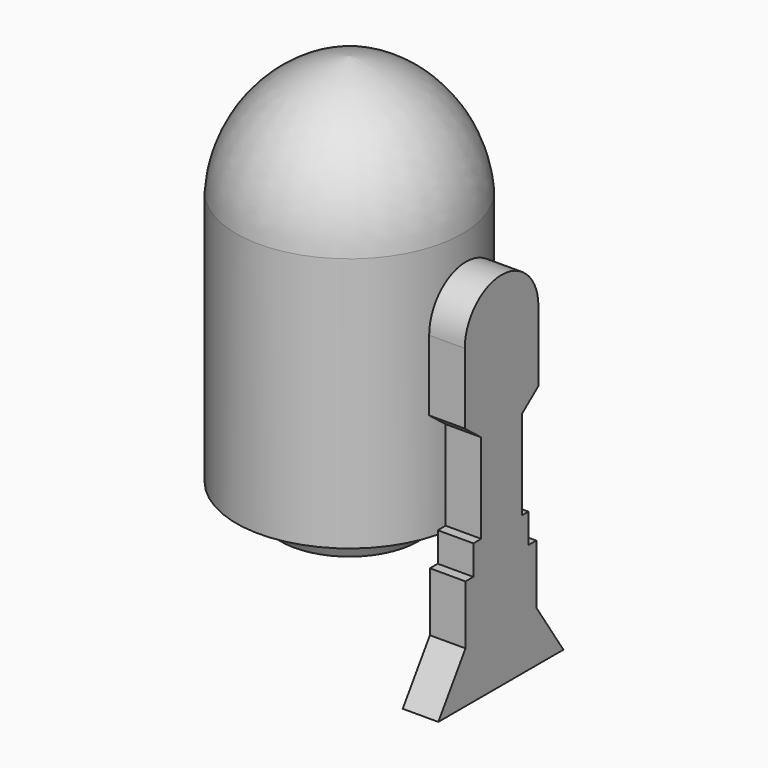
from build123d import *

# Parameters (mm, degrees)
F4_DEPTH = 8.8


with BuildPart() as f1:
    # F0 (on Front) → F1 (revolve)
    with BuildSketch(Plane.XZ):
        with BuildLine():
            ThreePointArc((27.9495026916, 0), (19.2278922615, 19.7592115619), (0, 29.5969495755))
            Line((0, 29.5969495755), (0, -70.4030504245))
            Line((0, -70.4030504245), (16.9765111059, -70.5251395702))
            Line((16.9765111059, -70.5251395702), (20.9008958191, -63.0331337452))
            Line((20.9008958191, -63.0331337452), (27.9495026916, -63.0331337452))
            Line((27.9495026916, -63.0331337452), (27.9495026916, 0))
        make_face()
    revolve(axis=Axis((0, 0, -20.4030504245), (0, 0, -1)))


with BuildPart() as f4:
    # F3 (on offset) → F4 (new body)
    with BuildSketch(Plane.YZ.offset(28)):
        with BuildLine():
            Line((-10.345963412, -17.8559850901), (-10.345963412, -35.3041645139))
            Line((-10.345963412, -35.3041645139), (-5.2661128575, -39.2796974629))
            Line((-5.2661128575, -39.2796974629), (-5.2661128575, -61.3659974188))
            Line((-5.2661128575, -61.3659974188), (-7.6956056291, -61.3659974188))
            Line((-7.6956056291, -61.3659974188), (-7.6956056291, -68.6544794589))
            Line((-7.6956056291, -68.6544794589), (-10.1250984007, -68.6544794589))
            Line((-10.1250984007, -68.6544794589), (-10.1250984007, -83.2314360887))
            Line((-10.1250984007, -83.2314360887), (-18.5178943211, -95.8206299692))
            Line((-18.5178943211, -95.8206299692), (20.1331399148, -95.8206299692))
            Line((20.1331399148, -95.8206299692), (11.7403439945, -83.2314360887))
            Line((11.7403439945, -83.2314360887), (11.7403439945, -68.6544794589))
            Line((11.7403439945, -68.6544794589), (9.3108512228, -68.6544794589))
            Line((9.3108512228, -68.6544794589), (9.3108512228, -61.3659974188))
            Line((9.3108512228, -61.3659974188), (7.3230810231, -61.3659974188))
            Line((7.3230810231, -61.3659974188), (7.3230810231, -39.2796974629))
            Line((7.3230810231, -39.2796974629), (12.4029315775, -35.3041645139))
            Line((12.4029315775, -35.3041645139), (12.4029315775, -17.8559850901))
            ThreePointArc((12.4029315775, -17.8559850901), (1.0284840828, -6.4815375954), (-10.345963412, -17.8559850901))
        make_face()
    extrude(amount=F4_DEPTH)


solid = Compound([f1.part, f4.part])
